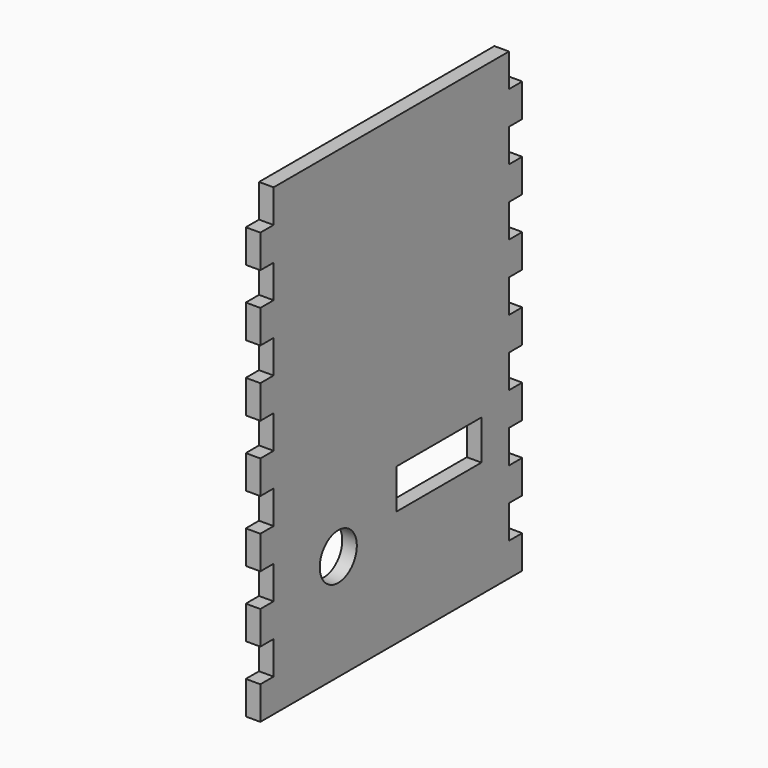
from build123d import *

# Parameters (mm, degrees)
F0_W     = 125.476
F0_H     = 177.8
F1_DEPTH = 5.588
F2_W     = 6.35
F2_H     = 12.7
F3_DEPTH = 25.4
F4_R     = 8.89
F5_DEPTH = 25.4
F6_W     = 40.64
F6_H     = 15.24
F7_DEPTH = 25.4


# Not quite as in the source:
# - a pattern or mirror of a feature is missing from the dataset's text; its kind, count and spacing are read off the source's solid


with BuildPart() as f1:
    # F0 (on Right) → F1 (new body)
    with BuildSketch(Plane.YZ):
        Rectangle(F0_W, F0_H)
    extrude(amount=F1_DEPTH)

    # F2 (on Right) → F3 (cut)
    with BuildSketch(Plane.YZ):
        with Locations((59.563, 82.55)):
            Rectangle(F2_W, F2_H)
        with Locations((59.563, 57.15)):
            Rectangle(F2_W, F2_H)
        with Locations((59.563, 31.75)):
            Rectangle(F2_W, F2_H)
        with Locations((59.563, 6.35)):
            Rectangle(F2_W, F2_H)
        with Locations((59.563, -19.05)):
            Rectangle(F2_W, F2_H)
        with Locations((59.563, -44.45)):
            Rectangle(F2_W, F2_H)
        with Locations((59.563, -69.85)):
            Rectangle(F2_W, F2_H)
    f3 = extrude(amount=F3_DEPTH, mode=Mode.SUBTRACT)

    # F3_copies: F3 across plane
    add(f3.mirror(Plane(origin=(0, 0, 0), x_dir=(0, 0, -1), z_dir=(0, -1, 0))), mode=Mode.SUBTRACT)

    # F4 (on Right) → F5 (cut)
    with BuildSketch(Plane.YZ):
        with Locations((-25.4, -48.26)):
            Circle(F4_R)
    extrude(amount=F5_DEPTH, mode=Mode.SUBTRACT)

    # F6 (on Right) → F7 (cut)
    with BuildSketch(Plane.YZ):
        with Locations((22.86, -36.83)):
            Rectangle(F6_W, F6_H)
    extrude(amount=F7_DEPTH, mode=Mode.SUBTRACT)


solid = f1.part
